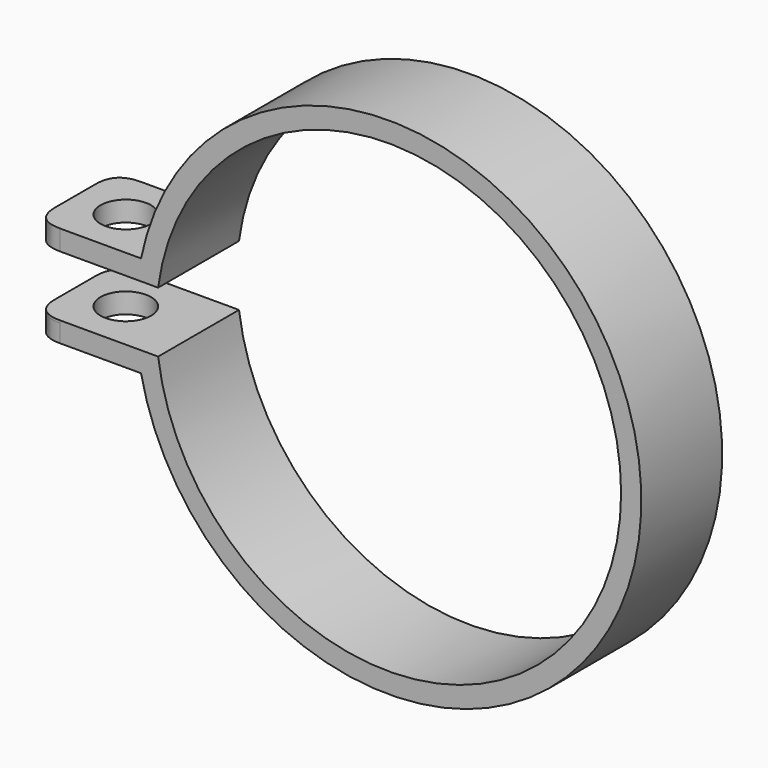
from build123d import *

# Parameters (mm, degrees)
F1_DEPTH    = 10
F2_T1_DEPTH = 29
F2_T3_DEPTH = 29
F3_R        = 5
F4_DEPTH    = 25.4


# Not quite as in the source:
# - a fillet or chamfer that OpenCascade refuses, or shapes differently, is made with other operations: its cross-section is extruded or revolved along the edge and cut away or added


with BuildPart() as f1:
    # F0 (on Front) → F1 (new body, symmetric)
    with BuildSketch(Plane.XZ):
        with BuildLine():
            Line((-70, -10), (-48.9897948557, -10))
            ThreePointArc((-48.9897948557, -10), (50, 0), (-48.9897948557, 10))
            Line((-48.9897948557, 10), (-70, 10))
            Line((-70, 10), (-70, 6))
            Line((-70, 6), (-45.607017004, 6))
            ThreePointArc((-45.607017004, 6), (46, 0), (-45.607017004, -6))
            Line((-45.607017004, -6), (-70, -6))
            Line((-70, -6), (-70, -10))
        make_face()
    extrude(amount=F1_DEPTH, both=True)

    # F2: fillet of radius 5 on 4 edges, made by hand

    # F2_s2 → F2_t1 (cut)
    with BuildSketch(Plane.XY.offset(-6.5)):
        with BuildLine():
            add(Edge.make_bspline(
                [(-70, 5), (-70, 10), (-65, 10)],
                knots=[0, 0, 0, 1, 1, 1], degree=2, weights=[1, 1, 1]))
            Line((-65, 10), (-70, 10))
            Line((-70, 10), (-70, 5))
        make_face()
        with BuildLine():
            add(Edge.make_bspline(
                [(-70, -5), (-70, -10), (-65, -10)],
                knots=[0, 0, 0, 1, 1, 1], degree=2, weights=[1, 1, 1]))
            Line((-65, -10), (-70, -10))
            Line((-70, -10), (-70, -5))
        make_face()
    extrude(amount=F2_T1_DEPTH, mode=Mode.SUBTRACT)

    # F2_s4 → F2_t3 (cut)
    with BuildSketch(Plane.XY.offset(-22.5)):
        with BuildLine():
            add(Edge.make_bspline(
                [(-70, 5), (-70, 10), (-65, 10)],
                knots=[0, 0, 0, 1, 1, 1], degree=2, weights=[1, 1, 1]))
            Line((-65, 10), (-70, 10))
            Line((-70, 10), (-70, 5))
        make_face()
        with BuildLine():
            add(Edge.make_bspline(
                [(-65, -10), (-70, -10), (-70, -5)],
                knots=[0, 0, 0, 1, 1, 1], degree=2, weights=[1, 1, 1]))
            Line((-70, -5), (-70, -10))
            Line((-70, -10), (-65, -10))
        make_face()
    extrude(amount=F2_T3_DEPTH, mode=Mode.SUBTRACT)

    # F3 (on face) → F4 (cut)
    with BuildSketch(Plane.XY.offset(10)):
        with Locations((-60, 0)):
            Circle(F3_R)
    extrude(amount=-F4_DEPTH, mode=Mode.SUBTRACT)


solid = f1.part
